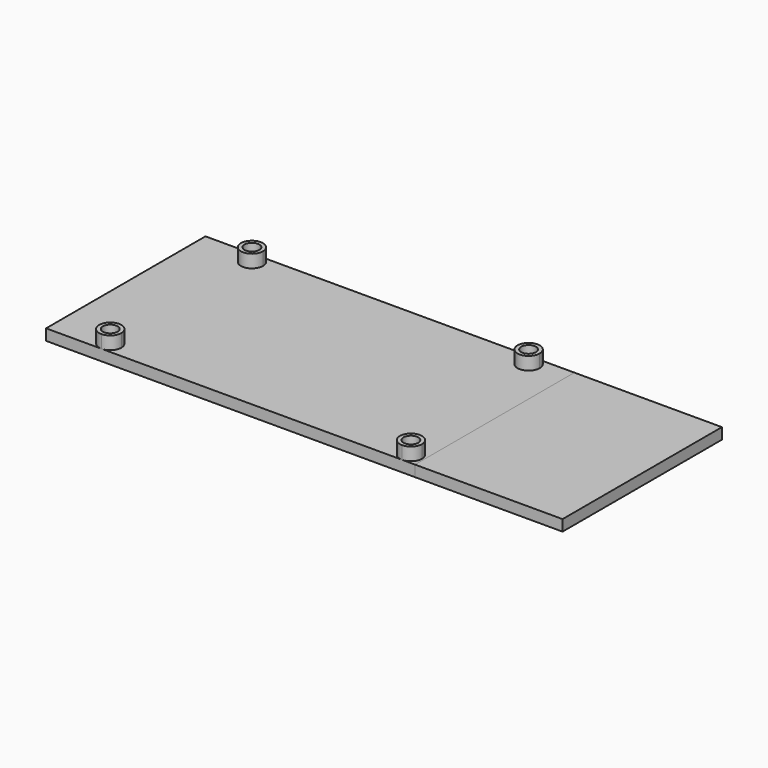
from build123d import *

# Parameters (mm, degrees)
F0_R        = 2
F1_DEPTH    = 6.5
F0_W        = 40
F0_H        = 54
F2_DEPTH    = 3
F3_E0_TOP_W = 100
F3_E0_TOP_H = 3
F4_DEPTH    = 54
F5_D        = 4


with BuildPart() as f1:
    # F0 (on Top) → F1 (new body)
    with BuildSketch(Plane.XY):
        with BuildLine():
            ThreePointArc((-32, -24), (-37.1213203436, -21.8786796564), (-35, -27))
            ThreePointArc((-35, -27), (-32.8786796564, -26.1213203436), (-32, -24))
        make_face()
        with Locations((-35, -24)):
            Circle(F0_R, mode=Mode.SUBTRACT)
    extrude(amount=F1_DEPTH)


with BuildPart() as f1b:
    # F0 (on Top) → F1, piece 2 (new body)
    with BuildSketch(Plane.XY):
        with BuildLine():
            ThreePointArc((-32, 24), (-32.8786796564, 26.1213203436), (-35, 27))
            ThreePointArc((-35, 27), (-37.1213203436, 21.8786796564), (-32, 24))
        make_face()
        with Locations((-35, 24)):
            Circle(F0_R, mode=Mode.SUBTRACT)
    extrude(amount=F1_DEPTH)


with BuildPart() as f1c:
    # F0 (on Top) → F1, piece 3 (new body)
    with BuildSketch(Plane.XY):
        with BuildLine():
            ThreePointArc((43, 24), (42.1213203436, 26.1213203436), (40, 27))
            ThreePointArc((40, 27), (37.8786796564, 21.8786796564), (43, 24))
        make_face()
        with Locations((40, 24)):
            Circle(F0_R, mode=Mode.SUBTRACT)
    extrude(amount=F1_DEPTH)


with BuildPart() as f1d:
    # F0 (on Top) → F1, piece 4 (new body)
    with BuildSketch(Plane.XY):
        with BuildLine():
            ThreePointArc((49.5, -24), (44.3786796564, -21.8786796564), (46.5, -27))
            ThreePointArc((46.5, -27), (48.6213203436, -26.1213203436), (49.5, -24))
        make_face()
        with Locations((46.5, -24)):
            Circle(F0_R, mode=Mode.SUBTRACT)
    extrude(amount=F1_DEPTH)


with BuildPart() as f2:
    # F0 (on Top) → F2 (new body)
    with BuildSketch(Plane.XY):
        with Locations((70, 0)):
            Rectangle(F0_W, F0_H)
    extrude(amount=F2_DEPTH)


with BuildPart() as f4:
    # F3_E0_top (on explicit) → F4 (new body)
    with BuildSketch(Plane(origin=(-50, -27, 0), x_dir=(1, 0, 0), z_dir=(0, -1, 0))):
        with Locations((50, 1.5)):
            Rectangle(F3_E0_TOP_W, F3_E0_TOP_H)
    extrude(amount=-F4_DEPTH)

    # F5 (through all)
    with Locations(Plane(origin=(0, 0, 0), x_dir=(1, 0, 0), z_dir=(0, 0, -1))):
        with Locations((40, -24), (46.5, 24), (-35, 24), (-35, -24)):
            Hole(F5_D / 2)


solid = Compound([f1.part, f1b.part, f1c.part, f1d.part, f2.part, f4.part])
